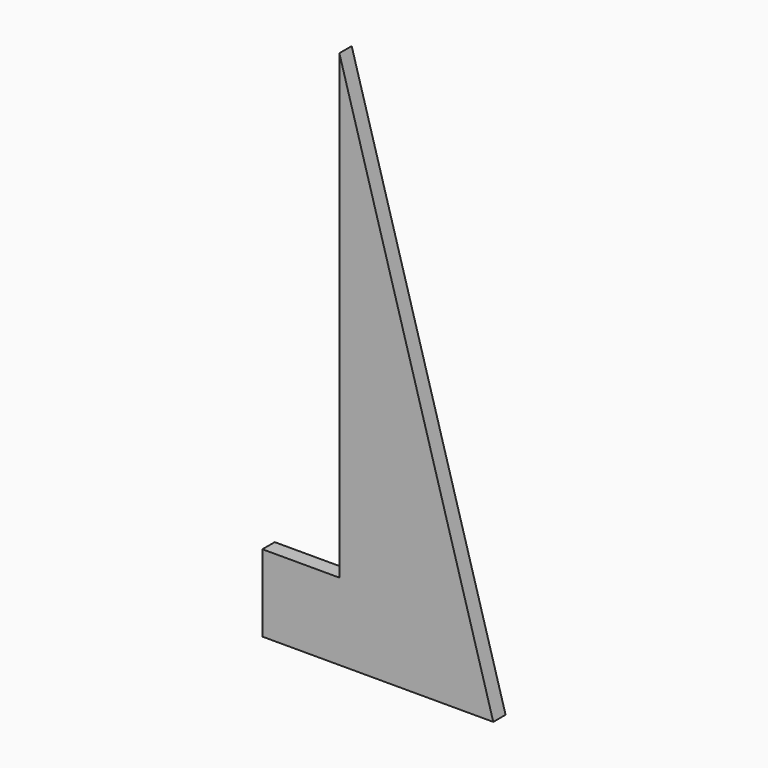
from build123d import *

# Parameters (mm, degrees)
F1_DEPTH = 5.08


# Not quite as in the source:
# - a feature names something its author has since deleted; it is built from what else it names


with BuildPart() as f1:
    # F0 (on Front) → F1 (new body)
    with BuildSketch(Plane.XZ):
        Polygon((0, 177.8), (0, 25.4), (-25.4, 25.4), (-25.4, 0), (50.8, 0), align=None)
    extrude(amount=F1_DEPTH)


solid = f1.part
